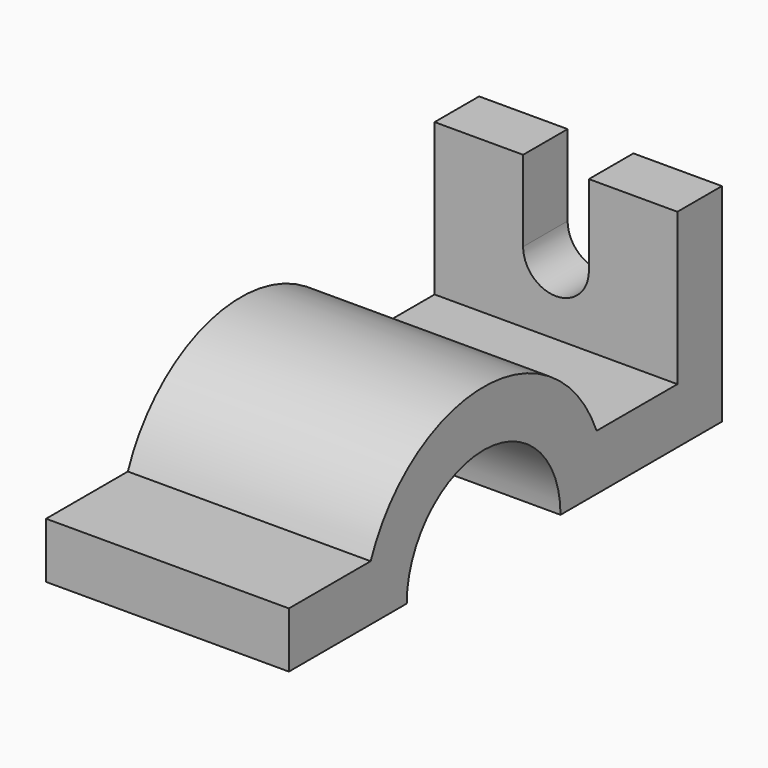
from build123d import *

# Parameters (mm, degrees)
F0_W     = 11
F0_H     = 30
F1_DEPTH = 24
F3_DEPTH = 30.3


with BuildPart() as f1:
    # F0 (on Right) → F1 (new body, symmetric)
    with BuildSketch(Plane.YZ):
        with BuildLine():
            Line((-48.1145605445, 0), (-30, 0))
            ThreePointArc((-30, 0), (-29.4730143031, 5.5983415304), (-27.9105714739, 11))
            Line((-27.9105714739, 11), (-48.1145605445, 11))
            Line((-48.1145605445, 11), (-48.1145605445, 0))
        make_face()
        with Locations((53.3854394555, 26)):
            Rectangle(F0_W, F0_H)
        with BuildLine():
            ThreePointArc((27.9105714739, 11), (29.4730143031, 5.5983415304), (30, 0))
            Line((30, 0), (58.8854394555, 0))
            Line((58.8854394555, 0), (58.8854394555, 11))
            Line((58.8854394555, 11), (47.8854394555, 11))
            Line((47.8854394555, 11), (27.9105714739, 11))
        make_face()
        with BuildLine():
            Line((15.4919333848, 11), (27.9105714739, 11))
            ThreePointArc((27.9105714739, 11), (0, 30), (-27.9105714739, 11))
            Line((-27.9105714739, 11), (-15.4919333848, 11))
            ThreePointArc((-15.4919333848, 11), (0, 19), (15.4919333848, 11))
        make_face()
        with BuildLine():
            Line((19, 0), (30, 0))
            ThreePointArc((30, 0), (29.4730143031, 5.5983415304), (27.9105714739, 11))
            Line((27.9105714739, 11), (15.4919333848, 11))
            ThreePointArc((15.4919333848, 11), (18.1017503893, 5.7729223833), (19, 0))
        make_face()
        with BuildLine():
            ThreePointArc((-27.9105714739, 11), (-29.4730143031, 5.5983415304), (-30, 0))
            Line((-30, 0), (-19, 0))
            ThreePointArc((-19, 0), (-18.1017503893, 5.7729223833), (-15.4919333848, 11))
            Line((-15.4919333848, 11), (-27.9105714739, 11))
        make_face()
    extrude(amount=F1_DEPTH, both=True)

    # F2 (on face) → F3 (cut)
    with BuildSketch(Plane(origin=(0, 58.8854394555, 0), x_dir=(-1, 0, 0), z_dir=(0, 1, 0))):
        with BuildLine():
            ThreePointArc((-6.5, 25), (0, 18.5), (6.5, 25))
            ThreePointArc((6.5, 25), (0, 31.5), (-6.5, 25))
        make_face()
        with BuildLine():
            ThreePointArc((-6.5, 25), (0, 31.5), (6.5, 25))
            Line((6.5, 25), (6.5, 41))
            Line((6.5, 41), (-6.5, 41))
            Line((-6.5, 41), (-6.5, 25))
        make_face()
    extrude(amount=-F3_DEPTH, mode=Mode.SUBTRACT)


solid = f1.part
